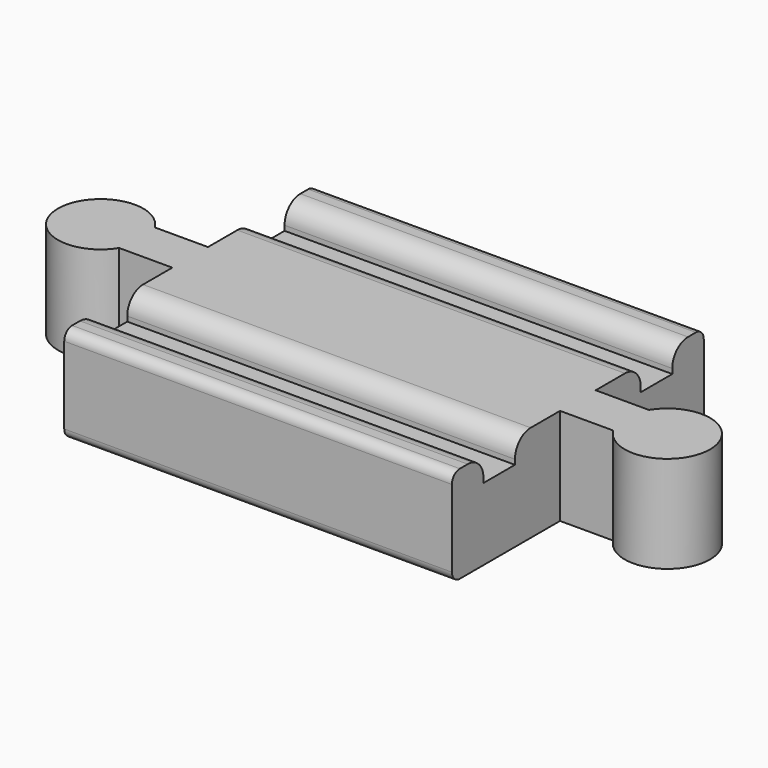
from build123d import *

# Parameters (mm, degrees)
F0_W     = 50
F0_H     = 40.6
F1_DEPTH = 12.5
F3_DEPTH = 12.5
F4_W     = 50
F4_H     = 5.08
F5_DEPTH = 3.175
F6_R     = 1.27
F7_R     = 2.54


# Not quite as in the source:
# - a pattern or mirror of a feature is missing from the dataset's text; its kind, count and spacing are read off the source's solid
# - a feature names something its author has since deleted; it is built from what else it names


with BuildPart() as f1:
    # F0 (on Top) → F1 (new body)
    with BuildSketch(Plane.XY):
        Rectangle(F0_W, F0_H)
    extrude(amount=F1_DEPTH)

    # F2 (on face) → F3 (join, through all)
    with BuildSketch(Plane.XY.offset(12.5)):
        with BuildLine():
            Line((25, -2.875), (31.8612501666, -2.875))
            ThreePointArc((31.8612501666, -2.875), (42.05, 0), (31.8612501666, 2.875))
            Line((31.8612501666, 2.875), (25, 2.875))
            Line((25, 2.875), (25, 0))
            Line((25, 0), (25, -2.875))
        make_face()
    f3 = extrude(amount=-F3_DEPTH)

    # F3_copies: F3 across plane
    add(f3.mirror(Plane(origin=(0, 0, 0), x_dir=(0, 0, -1), z_dir=(-1, 0, 0))))

    # F4 (on face) → F5 (cut)
    with BuildSketch(Plane.XY.offset(12.5)):
        with Locations((0, 12.68)):
            Rectangle(F4_W, F4_H)
    f5 = extrude(amount=-F5_DEPTH, mode=Mode.SUBTRACT)

    # F5_copies: F5 across plane
    add(f5.mirror(Plane(origin=(0, 0, 0), x_dir=(0, 0, -1), z_dir=(0, -1, 0))), mode=Mode.SUBTRACT)

    # F6
    f6_edges = [f1.edges().sort_by_distance(p)[0] for p in [
        (0, 20.3, 12.5),
        (0, -20.3, 12.5),
        (0, 20.3, 0),
        (0, -20.3, 0),
    ]]
    fillet(f6_edges, radius=F6_R)

    # F7
    f7_edges = [f1.edges().sort_by_distance(p)[0] for p in [
        (0, 15.22, 12.5),
        (0, 10.14, 12.5),
        (0, -10.14, 12.5),
        (0, -15.22, 12.5),
    ]]
    fillet(f7_edges, radius=F7_R)


solid = f1.part
